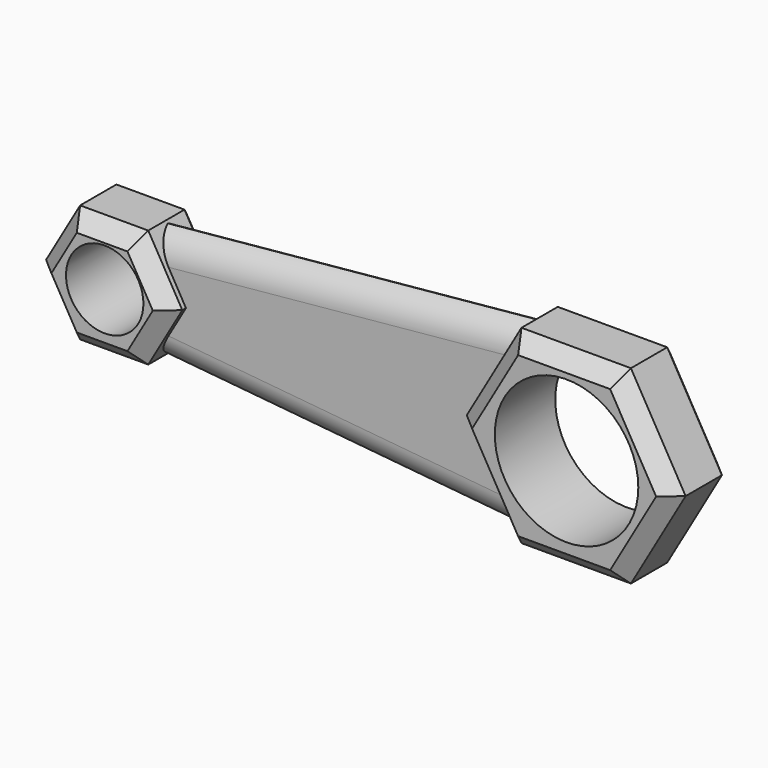
from build123d import *

# Parameters (mm, degrees)
F1_DEPTH    = 12.5
F2_DEPTH    = 12.5
F3_DEPTH    = 6
F5_R        = 12.8142300387
F4_R        = 23.7463809622
F8_T1_DEPTH = 174.1013942082
F8_T3_DEPTH = 174.1013942082
F9_SIZE     = 5
F9_2_SIZE   = 5


# Not quite as in the source:
# - a fillet or chamfer that OpenCascade refuses, or shapes differently, is made with other operations: its cross-section is extruded or revolved along the edge and cut away or added


with BuildPart() as f1:
    # F0 (on Front) → F1 (new body, symmetric)
    with BuildSketch(Plane.XZ):
        Polygon((18.1139551152, 31.3742905855), (-18.1139551152, 31.3742905855), (-36.2279102304, 0), (-18.1139551152, -31.3742905855), (18.1139551152, -31.3742905855), (36.2279102304, 0), align=None)
    extrude(amount=F1_DEPTH, both=True)

    # F7: sweep along a path in F7_path
    with BuildLine(Plane(origin=(18.1139551152, 12.5, -31.3742905855), x_dir=(0, 1, 0), z_dir=(0, 0, 1))) as f7_path:
        Line((0, 0), (-25, 0))
    # F4 (on face) → F7 (sweep, cut)
    with BuildSketch(Plane.XZ.offset(12.5)):
        with Locations((0.8038282976, 0.7768512587)):
            Circle(F4_R)
    sweep(path=f7_path.line, mode=Mode.SUBTRACT)

    # F9#2
    f9_2_edges = [f1.edges().sort_by_distance(p)[0] for p in [
        (27.170933, -12.5, -15.687145),
        (0, -12.5, -31.374291),
        (-27.170933, -12.5, -15.687145),
        (-27.170933, -12.5, 15.687145),
        (0, -12.5, 31.374291),
        (27.170933, -12.5, 15.687145),
        (27.170933, 12.5, 15.687145),
        (27.170933, 12.5, -15.687145),
        (0, 12.5, 31.374291),
        (-27.170933, 12.5, 15.687145),
        (-27.170933, 12.5, -15.687145),
        (0, 12.5, -31.374291),
    ]]
    chamfer(f9_2_edges, length=F9_2_SIZE)


with BuildPart() as f2:
    # F0 (on Front) → F2 (new body, symmetric)
    with BuildSketch(Plane.XZ):
        Polygon((-130.3748040067, 0), (-141.6485234433, 19.5266548544), (-164.1959623164, 19.5266548544), (-175.469681753, 0), (-164.1959623164, -19.5266548544), (-141.6485234433, -19.5266548544), align=None)
    extrude(amount=F2_DEPTH, both=True)

    # F6: sweep along a path in F6_path
    with BuildLine(Plane(origin=(-164.1959623164, 12.5, 19.5266548544), x_dir=(0, 1, 0), z_dir=(0, 0, 1))) as f6_path:
        Line((0, 0), (-25, 0))
    # F5 (on face) → F6 (sweep, cut)
    with BuildSketch(Plane.XZ.offset(12.5)):
        with Locations((-152.0675271749, 1.010288368)):
            Circle(F5_R)
    sweep(path=f6_path.line, mode=Mode.SUBTRACT)

    # F9
    f9_edges = [f2.edges().sort_by_distance(p)[0] for p in [
        (-152.922243, -12.5, -19.526655),
        (-169.832822, -12.5, -9.763327),
        (-169.832822, -12.5, 9.763327),
        (-152.922243, -12.5, 19.526655),
        (-136.011664, -12.5, -9.763327),
        (-136.011664, -12.5, 9.763327),
        (-152.922243, 12.5, -19.526655),
        (-169.832822, 12.5, -9.763327),
        (-169.832822, 12.5, 9.763327),
        (-152.922243, 12.5, 19.526655),
        (-136.011664, 12.5, 9.763327),
        (-136.011664, 12.5, -9.763327),
    ]]
    chamfer(f9_edges, length=F9_SIZE)


with BuildPart() as f3:
    # F0 (on Front) → F3 (new body, symmetric)
    with BuildSketch(Plane.XZ):
        Polygon((-36.2279102304, 0), (-18.1139551152, 31.3742905855), (-141.6485234433, 19.5266548544), (-130.3748040067, 0), (-141.6485234433, -19.5266548544), (-18.1139551152, -31.3742905855), align=None)
    extrude(amount=F3_DEPTH, both=True)

    # F8: fillet of radius 10 on 4 edges, made by hand

    # F8_s2 → F8_t1 (cut)
    with BuildSketch(Plane(origin=(-163.3877054019, 0, 15.669767926), x_dir=(0, 1, 0), z_dir=(0.9954325583, 0, -0.0954673862))):
        with BuildLine():
            ThreePointArc((-4, -32.960282292), (3.0710678119, -30.0313501039), (6, -22.960282292))
            Line((6, -22.960282292), (6, -32.960282292))
            Line((6, -32.960282292), (-4, -32.960282292))
        make_face()
        with BuildLine():
            ThreePointArc((4, -32.960282292), (-3.0710678119, -30.0313501039), (-6, -22.960282292))
            Line((-6, -22.960282292), (-6, -32.960282292))
            Line((-6, -32.960282292), (4, -32.960282292))
        make_face()
    extrude(amount=F8_T1_DEPTH, mode=Mode.SUBTRACT)

    # F8_s4 → F8_t3 (cut)
    with BuildSketch(Plane(origin=(9.9184908423, 0, 0.951237116), x_dir=(0, 1, 0), z_dir=(-0.9954325583, 0, -0.0954673862))):
        with BuildLine():
            ThreePointArc((4, -32.960282292), (-3.0710678119, -30.0313501039), (-6, -22.960282292))
            Line((-6, -22.960282292), (-6, -32.960282292))
            Line((-6, -32.960282292), (4, -32.960282292))
        make_face()
        with BuildLine():
            ThreePointArc((-4, -32.960282292), (3.0710678119, -30.0313501039), (6, -22.960282292))
            Line((6, -22.960282292), (6, -32.960282292))
            Line((6, -32.960282292), (-4, -32.960282292))
        make_face()
    extrude(amount=F8_T3_DEPTH, mode=Mode.SUBTRACT)


solid = Compound([f1.part, f2.part, f3.part])
